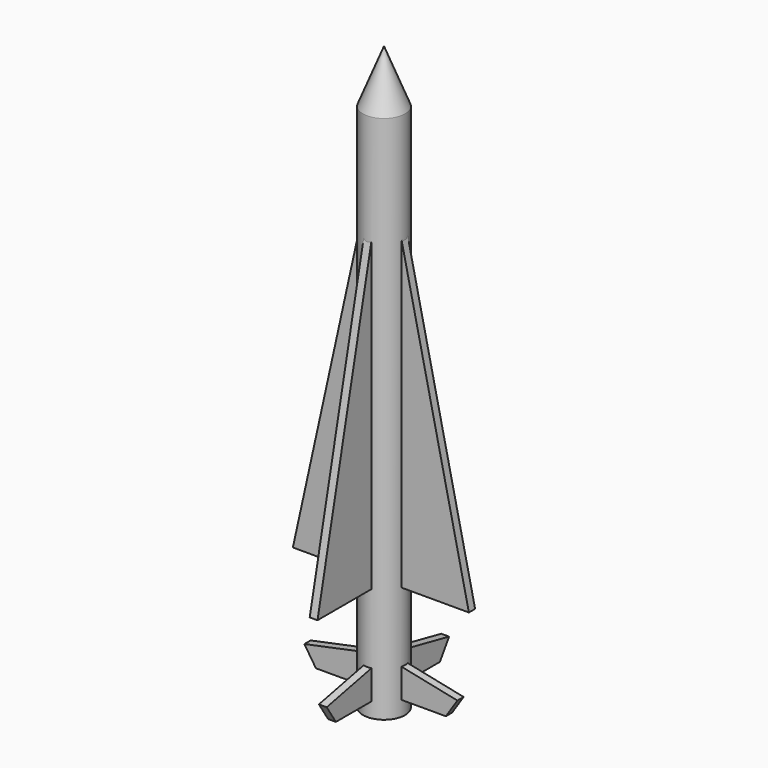
from build123d import *

# Parameters (mm, degrees)
F3_DEPTH     = 0.2
F4_COUNT     = 4
F7_DEPTH     = 10.0694444444
F8_T4_ANGLE  = 140.6790411595
F8_S5_R      = 0.2
F8_T6_DEPTH  = 4
F8_T10_ANGLE = 140.6790411595
F8_S11_R     = 0.2
F8_T12_DEPTH = 4


# Not quite as in the source:
# - a fillet or chamfer that OpenCascade refuses, or shapes differently, is made with other operations: its cross-section is extruded or revolved along the edge and cut away or added


with BuildPart() as f1:
    # F0 (on Front) → F1 (revolve)
    with BuildSketch(Plane.XZ):
        Polygon((0, 29.8611111111), (0, 0), (1.0763888889, 0), (1.0763888889, 27.1527777778), align=None)
    revolve(axis=Axis((0, 0, 14.9305555556), (0, 0, 1)))

    # F2 (on Front) → F3 (join, symmetric)
    with BuildSketch(Plane.XZ):
        Polygon((0, 2.4840856481), (0, 0.7638888889), (3.3333333333, 0.7638888889), (3.9236111111, 1.6666666667), (0.4, 2.4007523148), align=None)
        Polygon((0, 26.351010101), (0, 2.4840856481), (0.4, 2.4007523148), (0.4, 5.8333333333), (4.5138888889, 5.8333333333), align=None)
    extrude(amount=F3_DEPTH, both=True)

    # F4: F1 ×4 about axis
    f4_axis = Axis((0, 0, 0), (0, 0, 1))


with BuildPart() as f1_1:
    add(f1.part)
    for i in range(1, F4_COUNT):
        add(f1.part.rotate(f4_axis, i * 360 / F4_COUNT))

    # F6 (on offset) → F7 (join)
    with BuildSketch(Plane.XY.offset(6)):
        with BuildLine():
            Line((-0.7071923595, -0.424349647), (-0.9025432388, -0.6197005263))
            ThreePointArc((-0.9025432388, -0.6197005263), (-0.9025432388, -0.9025432388), (-0.6197005263, -0.9025432388))
            Line((-0.6197005263, -0.9025432388), (-0.424349647, -0.7071923595))
            Line((-0.424349647, -0.7071923595), (-0.7071923595, -0.424349647))
        make_face()
    extrude(amount=F7_DEPTH)

    # F8: chamfer of 0.25 x 0.4330127019 on 2 edges, made by hand


with BuildPart() as f8_tool2:
    # F8_s3 → F8_t4 (revolve)
    with BuildSketch(Plane(origin=(0, 0, 0), x_dir=(0, 0, 1), z_dir=(0.4279813655, 0.9037875584, 0))):
        with BuildLine():
            Line((16.5174571463, -1.0677286349), (16.0544444444, -1.3350491429))
            Line((16.0544444444, -1.3350491429), (16.0457841904, -1.3350491429))
            ThreePointArc((16.0457841904, -1.3350491429), (16.0607841904, -1.2057190159), (16.0607841904, -1.0763888889))
            Line((16.0607841904, -1.0763888889), (16.0694444444, -1.0677286349))
            ThreePointArc((16.0694444444, -1.0677286349), (16.2934507954, -1.0677286349), (16.5174571463, -1.0590683808))
            Line((16.5174571463, -1.0590683808), (16.5174571463, -1.0677286349))
        make_face()
    revolve(axis=Axis((0, 0, 16.0694444444), (0, 0, 1)), revolution_arc=F8_T4_ANGLE)

    # F8_s5 → F8_t6 (intersect, symmetric)
    with BuildSketch(Plane.XY.offset(16.1)):
        with Locations((-0.7611218825, -0.7611218825)):
            Circle(F8_S5_R)
    extrude(amount=F8_T6_DEPTH, both=True, mode=Mode.INTERSECT)


with BuildPart() as f1_2:
    add(f1_1.part)

    # F8_t1: union F8_tool2
    add(f8_tool2.part)


with BuildPart() as f8_tool8:
    # F8_s9 → F8_t10 (revolve)
    with BuildSketch(Plane(origin=(0, 0, 0), x_dir=(0, 0, 1), z_dir=(0.4279813655, 0.9037875584, 0))):
        with BuildLine():
            Line((5.5519872981, -1.0677286349), (6.015, -1.3350491429))
            Line((6.015, -1.3350491429), (6.023660254, -1.3350491429))
            ThreePointArc((6.023660254, -1.3350491429), (6.008660254, -1.2057190159), (6.008660254, -1.0763888889))
            Line((6.008660254, -1.0763888889), (6, -1.0677286349))
            ThreePointArc((6, -1.0677286349), (5.7759936491, -1.0677286349), (5.5519872981, -1.0590683808))
            Line((5.5519872981, -1.0590683808), (5.5519872981, -1.0677286349))
        make_face()
    revolve(axis=Axis((0, 0, 6), (0, 0, 1)), revolution_arc=F8_T10_ANGLE)

    # F8_s11 → F8_t12 (intersect, symmetric)
    with BuildSketch(Plane.XY.offset(5.9)):
        with Locations((-0.7611218825, -0.7611218825)):
            Circle(F8_S11_R)
    extrude(amount=F8_T12_DEPTH, both=True, mode=Mode.INTERSECT)


with BuildPart() as f1_3:
    add(f1_2.part)

    # F8_t7: union F8_tool8
    add(f8_tool8.part)


solid = f1_3.part
